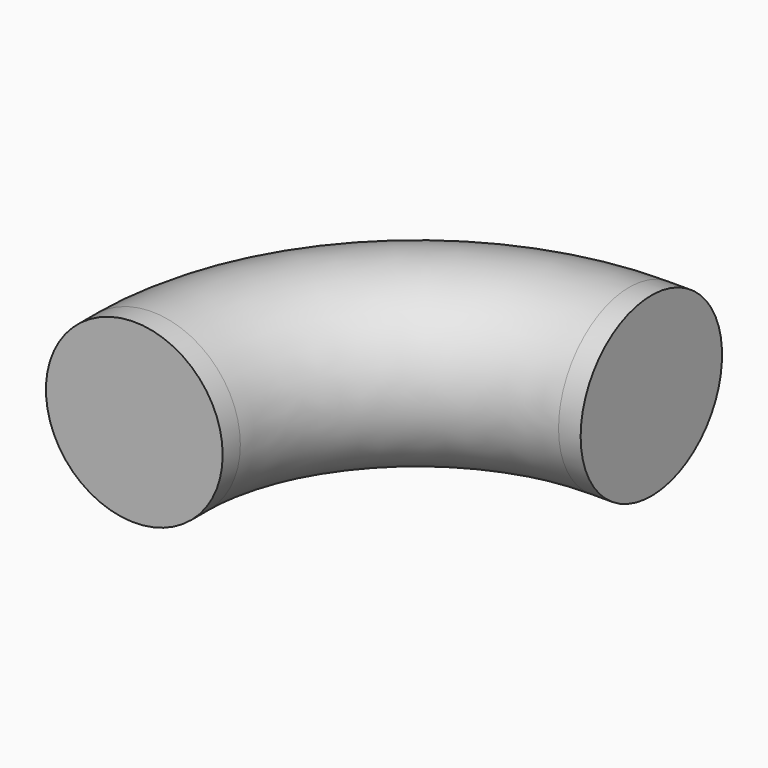
from build123d import *

# Parameters (mm, degrees)
F0_R     = 228.6
F3_DEPTH = 57.15
F4_DEPTH = 57.15


with BuildPart() as f2:
    # F2: sweep along a path in F1
    with BuildLine(Plane.XY) as f2_path:
        ThreePointArc((0, 457.2), (-323.2892203585, 323.2892203585), (-457.2, 0))
    # F0 (on Front) → F2 (sweep)
    with BuildSketch(Plane.XZ):
        with Locations((-685.8, 0)):
            Circle(F0_R)
    sweep(path=f2_path.line)

    # F3 (add): a face of the model
    f3_faces = [f2.faces().sort_by_distance(p)[0] for p in [
        (-685.8, 0, 0),
    ]]
    extrude(f3_faces, amount=F3_DEPTH)

    # F4 (add): a face of the model
    f4_faces = [f2.faces().sort_by_distance(p)[0] for p in [
        (0, 685.8, 0),
    ]]
    extrude(f4_faces, amount=F4_DEPTH)


solid = f2.part
